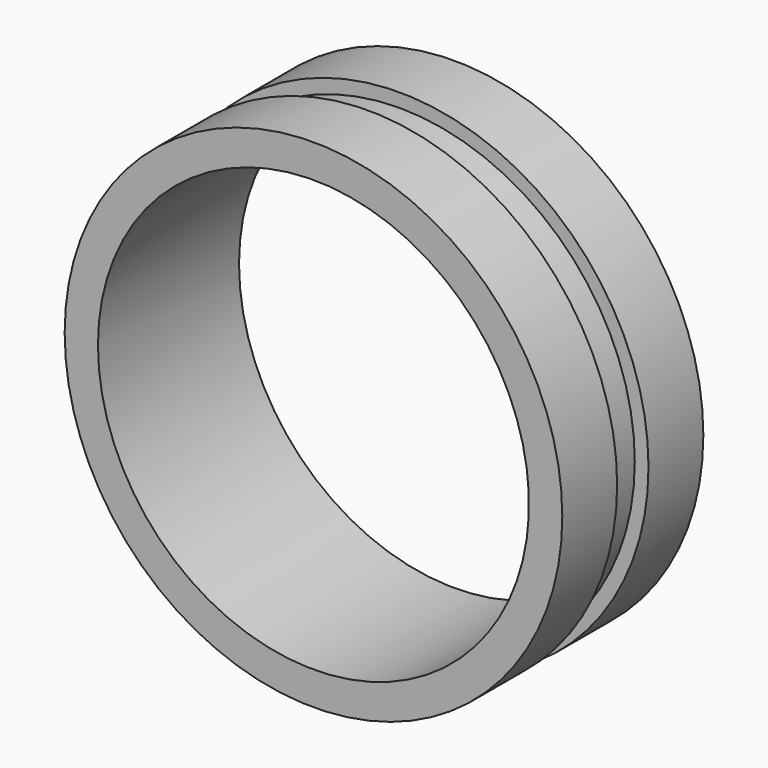
from build123d import *

# Parameters (mm, degrees)
F0_R     = 12
F1_DEPTH = 9
F2_R     = 12.7
F3_DEPTH = 3.5
F4_R     = 12.7
F4_R_2   = 12
F5_DEPTH = 3.5
F6_D     = 22


# Not quite as in the source:
# - a feature names something its author has since deleted; it is built from what else it names


with BuildPart() as f1:
    # F0 (on Front) → F1 (new body)
    with BuildSketch(Plane.XZ):
        with Locations((-29.9285538495, 19.7017099708)):
            Circle(F0_R)
    extrude(amount=F1_DEPTH)

    # F2 (on Front) → F3 (join)
    with BuildSketch(Plane.XZ):
        with Locations((-29.9285538495, 19.7017099708)):
            Circle(F2_R)
    extrude(amount=F3_DEPTH)

    # F4 (on face) → F5 (join)
    with BuildSketch(Plane.XZ.offset(9)):
        with Locations((-29.9285538495, 19.7017099708)):
            Circle(F4_R)
        with Locations((-29.9285538495, 19.7017099708)):
            Circle(F4_R_2, mode=Mode.SUBTRACT)
    extrude(amount=-F5_DEPTH)

    # F6 (through all)
    with Locations(Plane(origin=(0, 0, 0), x_dir=(1, 0, 0), z_dir=(0, 1, 0))):
        with Locations((-29.9285538495, -19.7017099708)):
            Hole(F6_D / 2)


solid = f1.part
